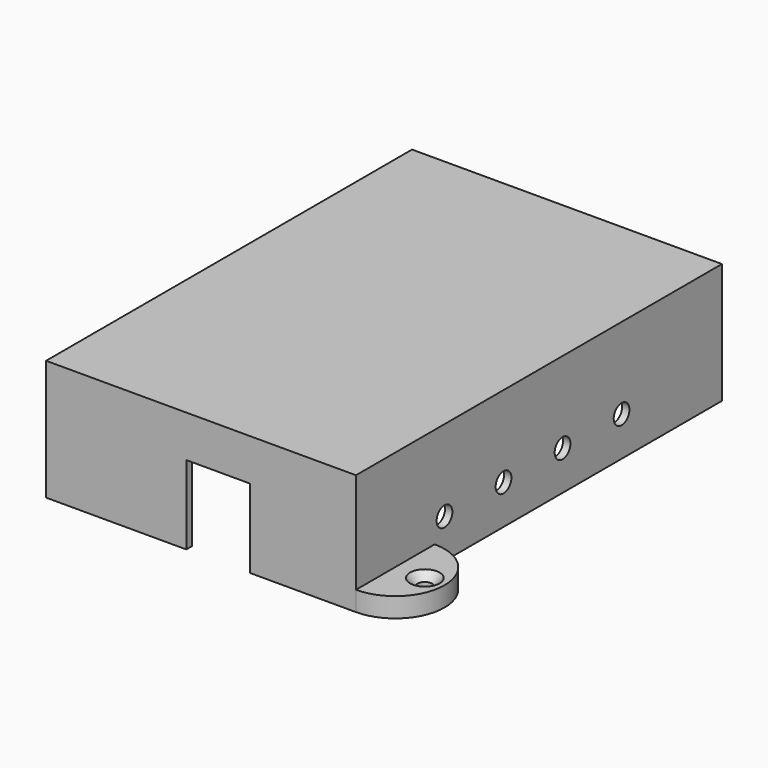
from build123d import *

# Parameters (mm, degrees)
F0_W      = 63
F0_H      = 93
F0_W_2    = 60
F0_H_2    = 90
F1_DEPTH  = 23
F2_W      = 13
F2_H      = 16
F3_DEPTH  = 25
F5_D      = 4
F5_DEPTH  = 12
F5_TIP    = 1.2017212381
F7_D      = 5
F7_DEPTH  = 12
F7_TIP    = 1.5021515476
F9_D      = 8
F9_DEPTH  = 12
F9_TIP    = 2.4034424761
F10_W     = 63
F10_H     = 93
F11_DEPTH = 1.5
F12_R     = 1.5
F13_DEPTH = 4
F14_SIZE  = 1.5


# Not quite as in the source:
# - a feature names something its author has since deleted; it is built from what else it names


with BuildPart() as f1:
    # F0 (on Top) → F1 (new body)
    with BuildSketch(Plane.XY):
        with Locations((30, 45)):
            Rectangle(F0_W, F0_H)
        with Locations((30, 45)):
            Rectangle(F0_W_2, F0_H_2, mode=Mode.SUBTRACT)
    extrude(amount=F1_DEPTH)

    # F2 (on face) → F3 (cut)
    with BuildSketch(Plane.XZ.offset(1.5)):
        with Locations((33.5, 8)):
            Rectangle(F2_W, F2_H)
    extrude(amount=-F3_DEPTH, mode=Mode.SUBTRACT)

    # F5
    with Locations(Plane.YZ.offset(61.5)):
        with Locations((51, 8), (66, 8), (36, 8), (21, 8)):
            Hole(F5_D / 2, depth=F5_DEPTH)
            with Locations((0, 0, -(F5_DEPTH + F5_TIP / 2))):  # 118° drill point
                Cone(0, F5_D / 2, F5_TIP, mode=Mode.SUBTRACT)

    # F7 (one way)
    with BuildSketch(Plane.XZ.offset(-90)):
        with Locations((13.5, 10), (38.5, 10)):
            Circle(F7_D / 2)
    extrude(amount=-F7_DEPTH, mode=Mode.SUBTRACT)
    with Locations(Plane.XZ.offset(-90)):
        with Locations((13.5, 10), (38.5, 10)):
            with Locations((0, 0, -(F7_DEPTH + F7_TIP / 2))):  # 118° drill point
                Cone(0, F7_D / 2, F7_TIP, mode=Mode.SUBTRACT)

    # F9
    with Locations(Plane(origin=(0, 91.5, 0), x_dir=(-1, 0, 0), z_dir=(0, 1, 0))):
        with Locations((-52.5, 16.5)):
            Hole(F9_D / 2, depth=F9_DEPTH)
            with Locations((0, 0, -(F9_DEPTH + F9_TIP / 2))):  # 118° drill point
                Cone(0, F9_D / 2, F9_TIP, mode=Mode.SUBTRACT)

    # F10 (on face) → F11 (join)
    with BuildSketch(Plane.XY.offset(23)):
        with Locations((30, 45)):
            Rectangle(F10_W, F10_H)
    extrude(amount=F11_DEPTH)

    # F12 (on face) → F13 (join)
    with BuildSketch(Plane(origin=(0, 0, 0), x_dir=(1, 0, 0), z_dir=(0, 0, -1))):
        with BuildLine():
            ThreePointArc((-1.5, -71.5), (-11.5, -81.5), (-1.5, -91.5))
            Line((-1.5, -91.5), (-1.5, -71.5))
        make_face()
        with Locations((-7.5, -81.5)):
            Circle(F12_R, mode=Mode.SUBTRACT)
        with BuildLine():
            Line((61.5, 1.5), (61.5, -18.5))
            ThreePointArc((61.5, -18.5), (71.5, -8.5), (61.5, 1.5))
        make_face()
        with Locations((67.5, -8.5)):
            Circle(F12_R, mode=Mode.SUBTRACT)
    extrude(amount=-F13_DEPTH)

    # F14
    f14_edges = [f1.edges().sort_by_distance(p)[0] for p in [
        (-9, 81.5, 4),
        (66, 8.5, 4),
    ]]
    chamfer(f14_edges, length=F14_SIZE)


solid = f1.part
